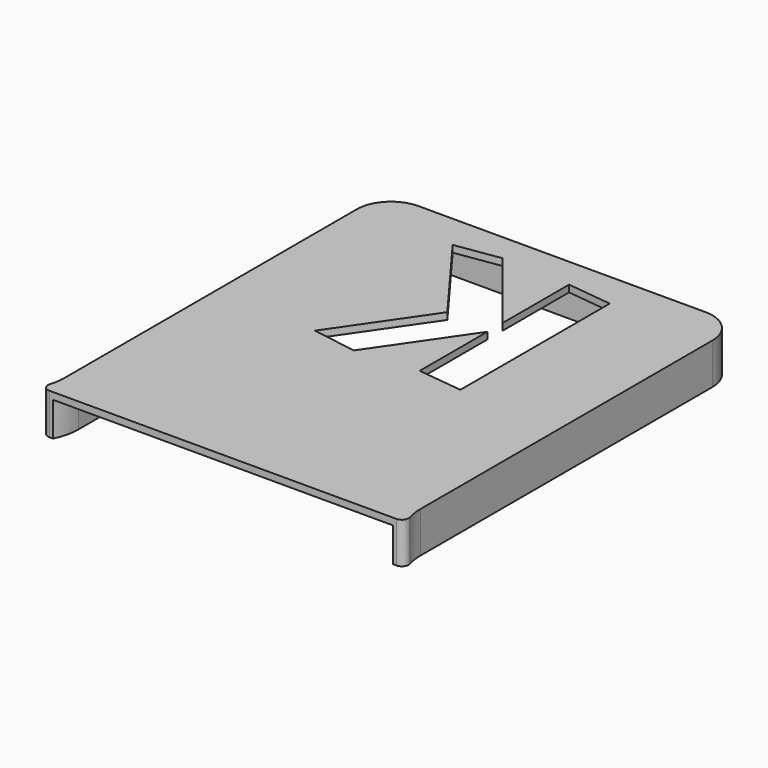
from build123d import *

# Parameters (mm, degrees)
F1_DEPTH = 1
F3_DEPTH = 6
F4_R     = 1
F5_R     = 5
F7_DEPTH = 12.5
F8_SCALE = 1.2


# Not quite as in the source:
# - a feature names something its author has since deleted; it is built from what else it names


with BuildPart() as f1:
    # F0 (on Top) → F1 (new body)
    with BuildSketch(Plane.XY):
        Polygon((24, 30), (-24, 30), (-24, -20.3061967343), (-24, -30), (24, -30), (24, -20.3061967343), align=None)
        Polygon((-24, -30), (-24, -20.3061967343), (-26.5, -30), align=None)
        Polygon((26.5, -30), (24, -20.3061967343), (24, -30), align=None)
    extrude(amount=F1_DEPTH)

    # F2 (on face) → F3 (join)
    with BuildSketch(Plane.XY.offset(1)):
        with BuildLine():
            Line((24, 30), (24, -26.4028457212))
            ThreePointArc((24, -26.4028457212), (24.2165144832, -28.2514541736), (24.8543383025, -30))
            Line((24.8543383025, -30), (26.8543383025, -30))
            ThreePointArc((26.8543383025, -30), (26.2165144832, -28.2514541736), (26, -26.4028457212))
            Line((26, -26.4028457212), (26, 32))
            Line((26, 32), (0, 32))
            Line((0, 32), (-26, 32))
            Line((-26, 32), (-26, -26.4028457212))
            ThreePointArc((-26, -26.4028457212), (-26.2165144832, -28.2514541736), (-26.8543383025, -30))
            Line((-26.8543383025, -30), (-24.8543383025, -30))
            ThreePointArc((-24.8543383025, -30), (-24.2165144832, -28.2514541736), (-24, -26.4028457212))
            Line((-24, -26.4028457212), (-24, 30))
            Line((-24, 30), (0, 30))
            Line((0, 30), (24, 30))
        make_face()
    extrude(amount=-F3_DEPTH)

    # F4
    f4_edges = [f1.edges().sort_by_distance(p)[0] for p in [
        (-26.854338, -30, -2),
        (26.854338, -30, -2),
    ]]
    fillet(f4_edges, radius=F4_R)

    # F5
    f5_edges = [f1.edges().sort_by_distance(p)[0] for p in [
        (24, 30, -2.5),
        (26, 32, -2),
        (-26, 32, -2),
        (-24, 30, -2.5),
    ]]
    fillet(f5_edges, radius=F5_R)


with BuildPart() as f7:
    # F6 (on face) → F7 (new body, symmetric)
    with BuildSketch(Plane(origin=(0, 0, 0), x_dir=(1, 0, 0), z_dir=(0, 0, -1))):
        Polygon((6.3998643309, -23.389915917), (11.8633387856, -22.7571071915), (11.8633387856, 0), (6.3998643309, -0.6328087254), (6.3998643309, -10.9478783381), (6.3998643309, -13.2169965655), align=None)
        Polygon((-1.9300751453, -23.6877743155), (6.3998643309, -13.2169965655), (6.3998643309, -10.9478783381), (-1.1277758749, 0), (-6.5578306463, -0.8743598687), (0.8998643309, -11.7196280624), (-7.3682154656, -22.865199178), align=None)
    extrude(amount=F7_DEPTH, both=True)


with BuildPart() as f7_1:
    # F8: moved
    add(f7.part.scale(F8_SCALE))


with BuildPart() as f7_2:
    # F9: moved
    add(f7_1.part.moved(Location((-3.1, -0.5, 0))))


with BuildPart() as f1_1:
    add(f1.part)

    # F10: cut F7
    add(f7_2.part, mode=Mode.SUBTRACT)


solid = f1_1.part
